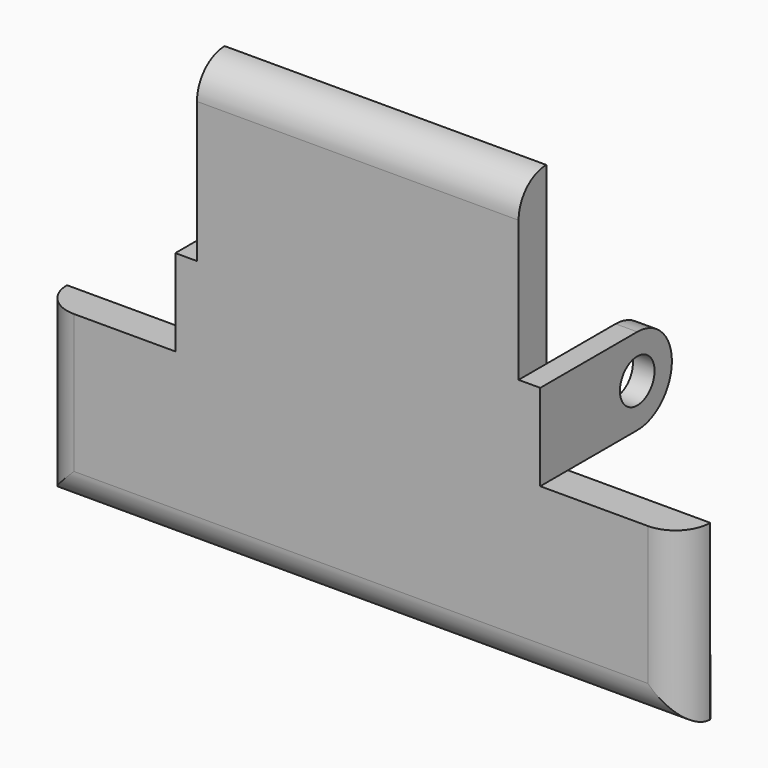
from build123d import *

# Parameters (mm, degrees)
F1_DEPTH     = 5.08
F2_R         = 5.07999
F3_R         = 3.175
F3_W         = 5.08
F3_H         = 12.7
F4_DEPTH     = 3.175
F5_R         = 3.175
F5_W         = 5.08
F5_H         = 12.7
F6_DEPTH     = 3.175
F7_W         = 94.3114114086
F7_H         = 7.62
F8_DEPTH     = 2.54
F9_T1_DEPTH  = 116.3084855321
F9_T6_DEPTH  = 29.6170741236
F9_T11_DEPTH = 29.6170741236


# Not quite as in the source:
# - a fillet or chamfer that OpenCascade refuses, or shapes differently, is made with other operations: its cross-section is extruded or revolved along the edge and cut away or added
# - a fillet or chamfer is up to 0.001 mm smaller than in the source, because OpenCascade refuses the exact size


with BuildPart() as f1:
    # F0 (on Front) → F1 (new body)
    with BuildSketch(Plane.XZ):
        Polygon((-23.1219715205, 38.3847513186), (-23.1219715205, 0), (-46.243943041, 0), (-46.243943041, -25.4), (48.0674683675, -25.4), (48.0674683675, 0), (24.0337341838, 0), (24.0337341838, 38.3847513186), align=None)
    extrude(amount=F1_DEPTH)

    # F2 (radius 5.08 in the source; OpenCascade refuses exactly that, so slightly less here)
    f2_edges = [f1.edges().sort_by_distance(p)[0] for p in [
        (-46.243943, -5.08, -12.7),
        (48.067468, -5.08, -12.7),
        (0.911763, -5.08, -25.4),
        (0.455881, -5.08, 38.384751),
    ]]
    fillet(f2_edges, radius=F2_R)

    # F3 (on face) → F4 (join)
    with BuildSketch(Plane(origin=(-23.1219715205, 0, 0), x_dir=(0, -1, 0), z_dir=(-1, 0, 0))):
        with BuildLine():
            Line((-12.7, 0), (0, 0))
            Line((0, 0), (0, 12.7))
            Line((0, 12.7), (-12.7, 12.7))
            ThreePointArc((-12.7, 12.7), (-19.05, 6.35), (-12.7, 0))
        make_face()
        with Locations((-12.7, 6.35)):
            Circle(F3_R, mode=Mode.SUBTRACT)
        with Locations((2.54, 6.35)):
            Rectangle(F3_W, F3_H)
    extrude(amount=F4_DEPTH)

    # F5 (on face) → F6 (join)
    with BuildSketch(Plane.YZ.offset(24.0337341838)):
        with BuildLine():
            Line((0, 12.7), (0, 0))
            Line((0, 0), (12.7, 0))
            ThreePointArc((12.7, 0), (19.05, 6.35), (12.7, 12.7))
            Line((12.7, 12.7), (0, 12.7))
        make_face()
        with Locations((12.7, 6.3747640323)):
            Circle(F5_R, mode=Mode.SUBTRACT)
        with Locations((-2.54, 6.35)):
            Rectangle(F5_W, F5_H)
    extrude(amount=F6_DEPTH)

    # F7 (on face) → F8 (join)
    with BuildSketch(Plane(origin=(0, 0, 0), x_dir=(-1, 0, 0), z_dir=(0, 1, 0))):
        with Locations((-0.9117626632, -21.59)):
            Rectangle(F7_W, F7_H)
    extrude(amount=F8_DEPTH)

    # F9: fillet of radius 5.08 on 3 edges, made by hand

    # F9_s2 → F9_t1 (cut)
    with BuildSketch(Plane.YZ.offset(-57.2424801028)):
        with BuildLine():
            ThreePointArc((-1e-05, -25.4), (1.8594061645, -23.5405901753), (2.54, -21.0005851753))
            Line((2.54, -21.0005851753), (2.54, -25.4))
            Line((2.54, -25.4), (-1e-05, -25.4))
        make_face()
    extrude(amount=F9_T1_DEPTH, mode=Mode.SUBTRACT)


with BuildPart() as f9_tool4:
    # F9_s5 → F9_t6 (new body)
    with BuildSketch(Plane.XY.offset(-36.3985370618)):
        with BuildLine():
            ThreePointArc((-46.243943041, -1e-05), (-44.3845332163, 1.8594061645), (-41.8445282163, 2.54))
            Line((-41.8445282163, 2.54), (-46.243943041, 2.54))
            Line((-46.243943041, 2.54), (-46.243943041, -1e-05))
        make_face()
    extrude(amount=F9_T6_DEPTH)

    split(bisect_by=Plane.XZ, keep=Keep.BOTTOM)


with BuildPart() as f1_1:
    add(f1.part)

    # F9_t3: cut F9_tool4
    add(f9_tool4.part, mode=Mode.SUBTRACT)


with BuildPart() as f9_tool9:
    # F9_s10 → F9_t11 (new body)
    with BuildSketch(Plane.XY.offset(-6.7814629382)):
        with BuildLine():
            ThreePointArc((43.6680535428, 2.54), (46.2080585428, 1.8594061645), (48.0674683675, -1e-05))
            Line((48.0674683675, -1e-05), (48.0674683675, 2.54))
            Line((48.0674683675, 2.54), (43.6680535428, 2.54))
        make_face()
    extrude(amount=-F9_T11_DEPTH)

    split(bisect_by=Plane.XZ, keep=Keep.BOTTOM)


with BuildPart() as f1_2:
    add(f1_1.part)

    # F9_t8: cut F9_tool9
    add(f9_tool9.part, mode=Mode.SUBTRACT)


solid = f1_2.part
